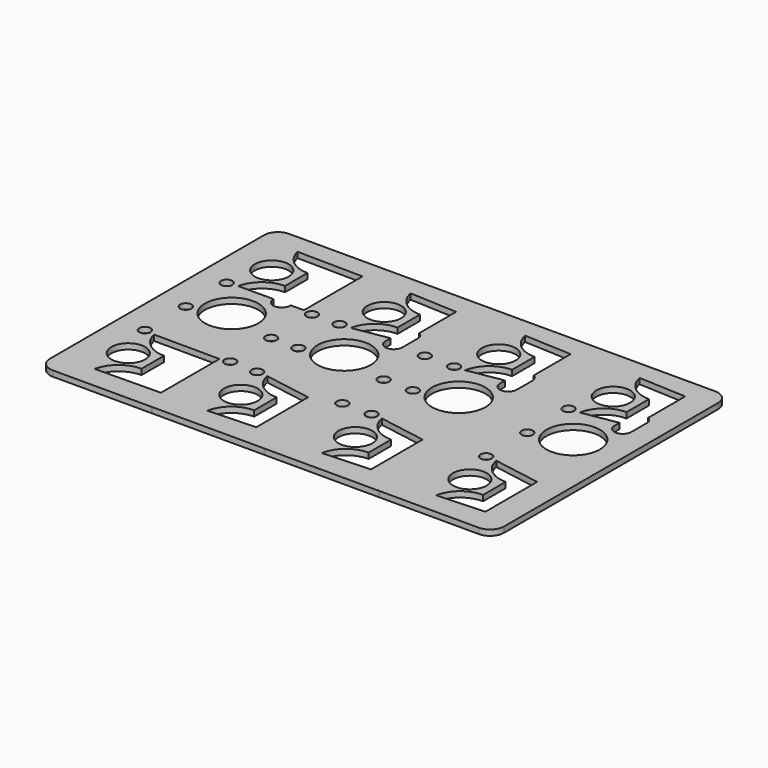
from build123d import *

# Parameters (mm, degrees)
F0_R     = 6
F0_R_2   = 2
F0_R_3   = 9.5
F1_DEPTH = 2
F2_R     = 5


# Not quite as in the source:
# - ends of sketch curves that miss each other by under 0.0002 mm in the source are joined


with BuildPart() as f1:
    # F0 (on Top) → F1 (new body)
    with BuildSketch(Plane.XY):
        Polygon((-23.8795465221, 51.1389637595), (-63.8795465221, 51.1389552037), (-63.8795465221, -53.8610447963), (-23.8795465221, -53.8610362327), (-23.3432798734, -53.8610447963), (16.1204534779, -53.861027669), (16.6553473944, -53.8610447963), (56.8043348949, -53.8610189589), (57.3406015435, -53.8610101337), (97.4896168807, -53.8610102485), (97.4896168807, 51.1389898663), (57.4896168808, 51.1389811639), (56.8043348949, 51.1389898663), (16.8043627316, 51.1389724616), (16.1204534779, 51.1389552037), (-23.1942645362, 51.138963906), align=None)
        with Locations((-48.9755360277, -32.7236170491)):
            Circle(F0_R, mode=Mode.SUBTRACT)
        with BuildLine():
            ThreePointArc((-40.2649926355, -27.7236170491), (-46.7743509608, -25.4265127742), (-50.3515408057, -19.5229421029))
            Line((-50.3515408057, -19.5229421029), (-27.0517710596, -19.6233615279))
            Line((-27.0517710596, -19.6233615279), (-27.0517710596, -45.6233615279))
            Line((-27.0517710596, -45.6233615279), (-50.3515408057, -45.9242919952))
            ThreePointArc((-50.3515408057, -45.9242919952), (-46.7743509608, -40.020721324), (-40.2649926355, -37.7236170491))
            Line((-40.2649926355, -37.7236170491), (-40.2649926355, -27.7236170491))
        make_face(mode=Mode.SUBTRACT)
        with Locations((-8.9769087599, -32.7076169273)):
            Circle(F0_R, mode=Mode.SUBTRACT)
        with BuildLine():
            ThreePointArc((-0.2663653677, -27.7076169273), (-6.7763425011, -25.3676442405), (-10.2489610341, -19.3846520981))
            Line((-10.2489610341, -19.3846520981), (6.5472276519, -22.2309003302))
            Line((6.5472276519, -22.2309003302), (6.5472276519, -45.2309003302))
            Line((6.5472276519, -45.2309003302), (-10.2489610341, -46.0305817564))
            ThreePointArc((-10.2489610341, -46.0305817564), (-6.7763425011, -40.047589614), (-0.2663653677, -37.7076169273))
            Line((-0.2663653677, -37.7076169273), (-0.2663653677, -27.7076169273))
        make_face(mode=Mode.SUBTRACT)
        with Locations((-54.0347284068, -19.0128381198)):
            Circle(F0_R_2, mode=Mode.SUBTRACT)
        with Locations((-23.7243646373, -19.0128381198)):
            Circle(F0_R_2, mode=Mode.SUBTRACT)
        with Locations((-14.0347284068, -19.1747317856)):
            Circle(F0_R_2, mode=Mode.SUBTRACT)
        with Locations((16.2756353627, -19.1747317856)):
            Circle(F0_R_2, mode=Mode.SUBTRACT)
        with Locations((31.7083453892, -32.7075822646)):
            Circle(F0_R, mode=Mode.SUBTRACT)
        with BuildLine():
            ThreePointArc((40.4188887821, -27.7075822646), (33.9089116483, -25.3676095781), (30.436293115, -19.3846174354))
            Line((30.436293115, -19.3846174354), (47.2324818011, -22.2308656676))
            Line((47.2324818011, -22.2308656676), (47.2324818011, -45.2308656676))
            Line((47.2324818011, -45.2308656676), (30.436293115, -46.0305470938))
            ThreePointArc((30.436293115, -46.0305470938), (33.9089116483, -40.0475549511), (40.4188887821, -37.7075822646))
            Line((40.4188887821, -37.7075822646), (40.4188887821, -27.7075822646))
        make_face(mode=Mode.SUBTRACT)
        with Locations((72.393430969, -32.7070186107)):
            Circle(F0_R, mode=Mode.SUBTRACT)
        with BuildLine():
            ThreePointArc((81.1039743612, -27.7070186107), (74.5943131753, -25.3674773264), (71.1213786947, -19.3851810893))
            Line((71.1213786947, -19.3851810893), (87.9175673808, -22.2314293214))
            Line((87.9175673808, -22.2314293214), (87.9175673808, -45.2314293214))
            Line((87.9175673808, -45.2314293214), (71.1213786947, -46.0288561321))
            ThreePointArc((71.1213786947, -46.0288561321), (74.5943131753, -40.046559895), (81.1039743612, -37.7070186107))
            Line((81.1039743612, -37.7070186107), (81.1039743612, -27.7070186107))
        make_face(mode=Mode.SUBTRACT)
        with Locations((26.6491530101, -19.1746971229)):
            Circle(F0_R_2, mode=Mode.SUBTRACT)
        with Locations((67.334434996, -19.1746971229)):
            Circle(F0_R_2, mode=Mode.SUBTRACT)
        with Locations((-54.0347284068, -0.8610447963)):
            Circle(F0_R_2, mode=Mode.SUBTRACT)
        with Locations((-41.5101771743, 3.8599752962)):
            Circle(F0_R_3, mode=Mode.SUBTRACT)
        with Locations((-23.7243646373, -0.8610447963)):
            Circle(F0_R_2, mode=Mode.SUBTRACT)
        with Locations((-54.0347284068, 17.2907485271)):
            Circle(F0_R_2, mode=Mode.SUBTRACT)
        with Locations((-23.7243646373, 17.2907485271)):
            Circle(F0_R_2, mode=Mode.SUBTRACT)
        with Locations((-14.0347284068, -0.8610447963)):
            Circle(F0_R_2, mode=Mode.SUBTRACT)
        with Locations((-1.5101771743, 3.8599752962)):
            Circle(F0_R_3, mode=Mode.SUBTRACT)
        with Locations((16.2756353627, -0.8610447963)):
            Circle(F0_R_2, mode=Mode.SUBTRACT)
        with Locations((-14.0347284068, 17.4526421929)):
            Circle(F0_R_2, mode=Mode.SUBTRACT)
        with Locations((16.2756353627, 17.4526421929)):
            Circle(F0_R_2, mode=Mode.SUBTRACT)
        with Locations((-48.9755360277, 31.0015274564)):
            Circle(F0_R, mode=Mode.SUBTRACT)
        with BuildLine():
            ThreePointArc((-40.2649926355, 36.0015274564), (-46.7743509608, 38.2986317313), (-50.3515408057, 44.2022024026))
            Line((-50.3515408057, 44.2022024026), (-27.0517710596, 43.9012719352))
            Line((-27.0517710596, 43.9012719352), (-27.0517710596, 17.9012719352))
            Line((-27.0517710596, 17.9012719352), (-31.7607614923, 17.8809767084))
            Line((-31.7607614923, 17.8809767084), (-31.7607756326, 17.7187155905))
            ThreePointArc((-31.7607756326, 17.7187155905), (-31.7603267926, 17.6887571457), (-31.7601771743, 17.6587957124))
            ThreePointArc((-31.7601771743, 17.6587957124), (-34.7601771743, 14.6587957124), (-37.7601771743, 17.6587957124))
            Line((-37.7601771743, 17.6587957124), (-37.7601771743, 17.8551198918))
            Line((-37.7601771743, 17.8551198918), (-50.3515408057, 17.8008525103))
            ThreePointArc((-50.3515408057, 17.8008525103), (-46.7743509608, 23.7044231815), (-40.2649926355, 26.0015274564))
            Line((-40.2649926355, 26.0015274564), (-40.2649926355, 36.0015274564))
        make_face(mode=Mode.SUBTRACT)
        with Locations((-8.9769087599, 30.9855273346)):
            Circle(F0_R, mode=Mode.SUBTRACT)
        with BuildLine():
            ThreePointArc((-0.2663653677, 35.9855273346), (-6.7763425011, 38.3255000213), (-10.2489610341, 44.3084921637))
            Line((-10.2489610341, 44.3084921637), (6.5472276519, 43.5088107375))
            Line((6.5472276519, 43.5088107375), (6.5472276519, 27.1076551873))
            ThreePointArc((6.5472276519, 27.1076551873), (7.7807259121, 26.0009361033), (8.2384500935, 24.4081920365))
            Line((8.2384500935, 24.4081920365), (8.2378516352, 17.5408218029))
            ThreePointArc((8.2378516352, 17.5408218029), (8.2383004752, 17.5108633581), (8.2384500935, 17.4809019247))
            ThreePointArc((8.2384500935, 17.4809019247), (5.2384500935, 14.4809019247), (2.2384500935, 17.4809019247))
            Line((2.2384500935, 17.4809019247), (2.2384500935, 19.7786539896))
            Line((2.2384500935, 19.7786539896), (-10.2489610341, 17.6625625054))
            ThreePointArc((-10.2489610341, 17.6625625054), (-6.7763425011, 23.6455546479), (-0.2663653677, 25.9855273346))
            Line((-0.2663653677, 25.9855273346), (-0.2663653677, 35.9855273346))
        make_face(mode=Mode.SUBTRACT)
        with Locations((26.6491530101, -0.8610101337)):
            Circle(F0_R_2, mode=Mode.SUBTRACT)
        with Locations((39.1737042426, 3.8600099589)):
            Circle(F0_R_3, mode=Mode.SUBTRACT)
        with Locations((26.6491530101, 17.4526768556)):
            Circle(F0_R_2, mode=Mode.SUBTRACT)
        with Locations((67.334434996, -0.8610101337)):
            Circle(F0_R_2, mode=Mode.SUBTRACT)
        with Locations((79.8589862285, 3.8600099589)):
            Circle(F0_R_3, mode=Mode.SUBTRACT)
        with Locations((67.334434996, 17.4526768556)):
            Circle(F0_R_2, mode=Mode.SUBTRACT)
        with Locations((31.7083453892, 30.9855619972)):
            Circle(F0_R, mode=Mode.SUBTRACT)
        with BuildLine():
            ThreePointArc((40.4188887821, 35.9855619972), (33.9089116483, 38.3255346838), (30.436293115, 44.3085268264))
            Line((30.436293115, 44.3085268264), (47.2324818011, 43.5088454002))
            Line((47.2324818011, 43.5088454002), (47.2324818011, 27.10768985))
            ThreePointArc((47.2324818011, 27.10768985), (48.4659800612, 26.000970766), (48.9237042426, 24.4082266992))
            Line((48.9237042426, 24.4082266992), (48.9231057843, 17.5408564655))
            ThreePointArc((48.9231057843, 17.5408564655), (48.9235546243, 17.5108980207), (48.9237042426, 17.4809365874))
            ThreePointArc((48.9237042426, 17.4809365874), (45.9237042426, 14.4809365874), (42.9237042426, 17.4809365874))
            Line((42.9237042426, 17.4809365874), (42.9237042426, 19.7786886523))
            Line((42.9237042426, 19.7786886523), (30.436293115, 17.6625971681))
            ThreePointArc((30.436293115, 17.6625971681), (33.9089116483, 23.6455893107), (40.4188887821, 25.9855619972))
            Line((40.4188887821, 25.9855619972), (40.4188887821, 35.9855619972))
        make_face(mode=Mode.SUBTRACT)
        with Locations((72.393430969, 30.9849983434)):
            Circle(F0_R, mode=Mode.SUBTRACT)
        with BuildLine():
            ThreePointArc((81.1039743612, 35.9849983434), (74.5943131753, 38.3245396276), (71.1213786947, 44.3068358648))
            Line((71.1213786947, 44.3068358648), (87.9175673808, 43.5094090541))
            Line((87.9175673808, 43.5094090541), (87.9175673808, 27.1071261961))
            ThreePointArc((87.9175673808, 27.1071261961), (89.151065641, 26.0004071121), (89.6087898224, 24.4076630453))
            Line((89.6087898224, 24.4076630453), (89.6081913641, 17.5402928116))
            ThreePointArc((89.6081913641, 17.5402928116), (89.6086402041, 17.5103343668), (89.6087898224, 17.4803729335))
            ThreePointArc((89.6087898224, 17.4803729335), (86.6087898224, 14.4803729335), (83.6087898224, 17.4803729335))
            Line((83.6087898224, 17.4803729335), (83.6087898224, 19.7792523062))
            Line((83.6087898224, 19.7792523062), (71.1213786947, 17.663160822))
            ThreePointArc((71.1213786947, 17.663160822), (74.5943131753, 23.6454570591), (81.1039743612, 25.9849983434))
            Line((81.1039743612, 25.9849983434), (81.1039743612, 35.9849983434))
        make_face(mode=Mode.SUBTRACT)
    extrude(amount=F1_DEPTH)

    # F2
    f2_edges = [f1.edges().sort_by_distance(p)[0] for p in [
        (-63.879547, 51.138955, 1),
        (97.489617, 51.13899, 1),
        (-63.879547, -53.861045, 1),
        (97.489617, -53.86101, 1),
    ]]
    fillet(f2_edges, radius=F2_R)


solid = f1.part
